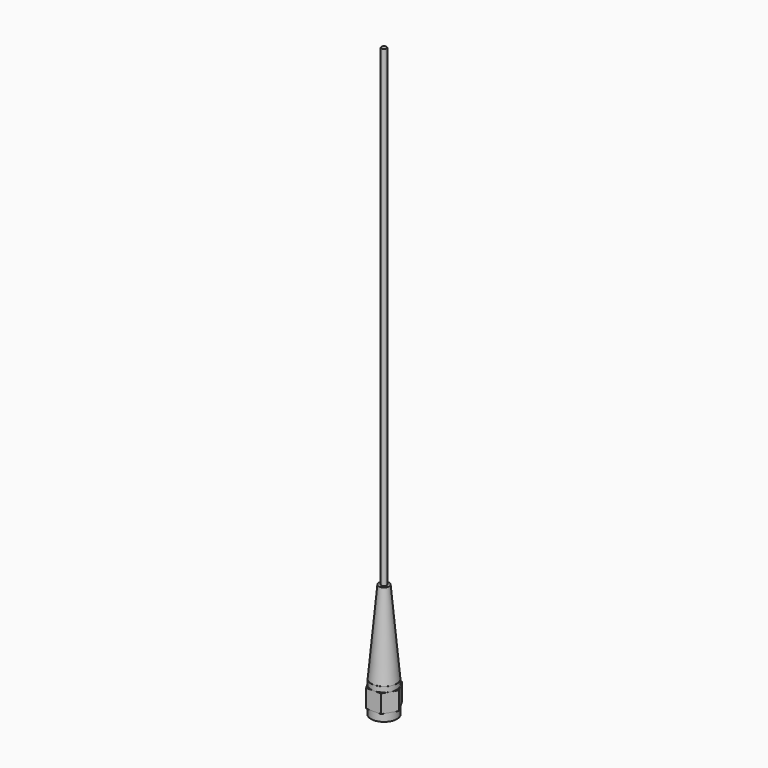
from build123d import *

# Parameters (mm, degrees)
F0_R      = 3.96875
F1_DEPTH  = 2.38125
F3_DEPTH  = 5.55625
F4_R      = 3.96875
F5_DEPTH  = 1.5875
F6_R      = 3.175
F7_DEPTH  = 3.175
F8_R      = 1.5875
F9_DEPTH  = 25.4
F12_R     = 0.79375
F13_DEPTH = 144.4625


# Not quite as in the source:
# - a length typed as a fraction of an inch, garbled in the dataset ("3 / 203.2 mm" for 3/8 in), is restored


with BuildPart() as f1:
    # F0 (on Top) → F1 (new body)
    with BuildSketch(Plane.XY):
        Circle(F0_R)
    extrude(amount=F1_DEPTH)

    # F2 (on face) → F3 (join)
    with BuildSketch(Plane.XY.offset(2.38125)):
        Polygon((2.2913588808, 3.96875), (-2.2913588808, 3.96875), (-4.5827177617, 0), (-2.2913588808, -3.96875), (2.2913588808, -3.96875), (4.5827177617, 0), align=None)
    extrude(amount=F3_DEPTH)

    # F4 (on face) → F5 (join)
    with BuildSketch(Plane.XY.offset(7.9375)):
        Circle(F4_R)
    extrude(amount=F5_DEPTH)

    # F6 (on face) → F7 (cut)
    with BuildSketch(Plane(origin=(0, 0, 0), x_dir=(1, 0, 0), z_dir=(0, 0, -1))):
        Circle(F6_R)
    extrude(amount=-F7_DEPTH, mode=Mode.SUBTRACT)

    # F8 (on face) → F9 (join)
    with BuildSketch(Plane.XY.offset(9.525)):
        Circle(F8_R)
    extrude(amount=F9_DEPTH)

    # F10 (on Front) → F11 (revolve)
    with BuildSketch(Plane.XZ):
        Polygon((1.5875, 34.925), (0, 34.925), (0, 9.525), (3.9187353296, 9.525), align=None)
    revolve(axis=Axis((0, 0, 9.525), (0, 0, 1)))

    # F12 (on face) → F13 (join)
    with BuildSketch(Plane.XY.offset(34.925)):
        Circle(F12_R)
    extrude(amount=F13_DEPTH)


solid = f1.part
